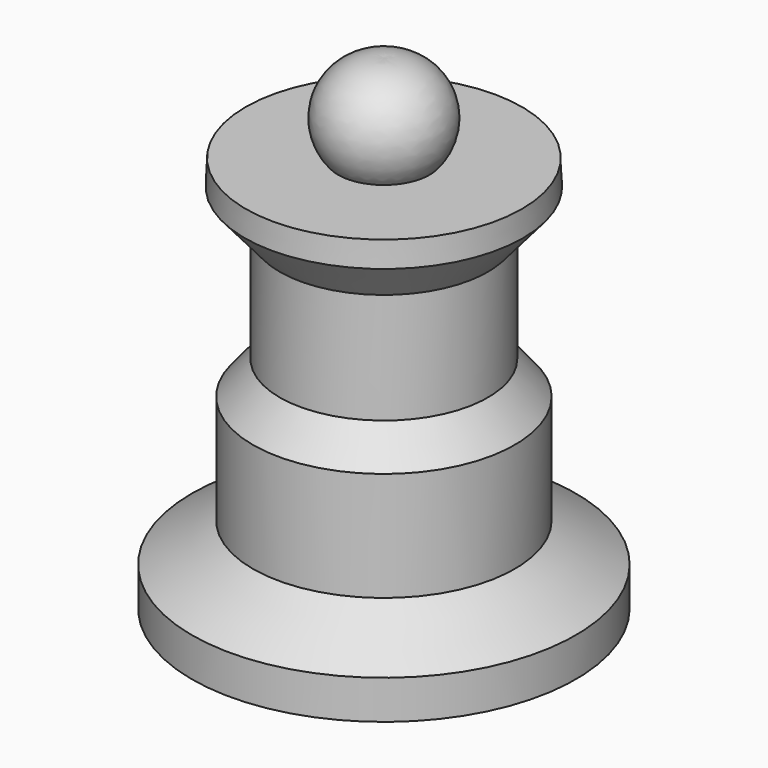
from build123d import *


# Not quite as in the source:
# - a feature names something its author has since deleted; it is built from what else it names


with BuildPart() as f1:
    # F0 (on Front) → F1 (revolve)
    with BuildSketch(Plane.XZ):
        with BuildLine():
            Line((-28.766008094, 0), (-28.766008094, -23.9662192762))
            Line((-28.766008094, -23.9662192762), (-42.1394705772, -32.4264727533))
            Line((-42.1394705772, -32.4264727533), (-42.1394705772, -40.9603528678))
            Line((-42.1394705772, -40.9603528678), (0, -40.9603528678))
            Line((0, -40.9603528678), (0, 65.5130892992))
            ThreePointArc((0, 65.5130892992), (-11.6659559175, 59.2375527161), (-10.0377807394, 46.0912249982))
            Line((-10.0377807394, 46.0912249982), (-30.3286965936, 46.1038053036))
            Line((-30.3286965936, 46.1038053036), (-30.560169369, 40.5484326184))
            Line((-30.560169369, 40.5484326184), (-22.8700842708, 31.5248221159))
            Line((-22.8700842708, 31.5248221159), (-22.8700842708, 7.2474917397))
            Line((-22.8700842708, 7.2474917397), (-28.766008094, 0))
        make_face()
    revolve(axis=Axis((0, 0, 12.2763682157), (0, 0, -1)))


solid = f1.part
